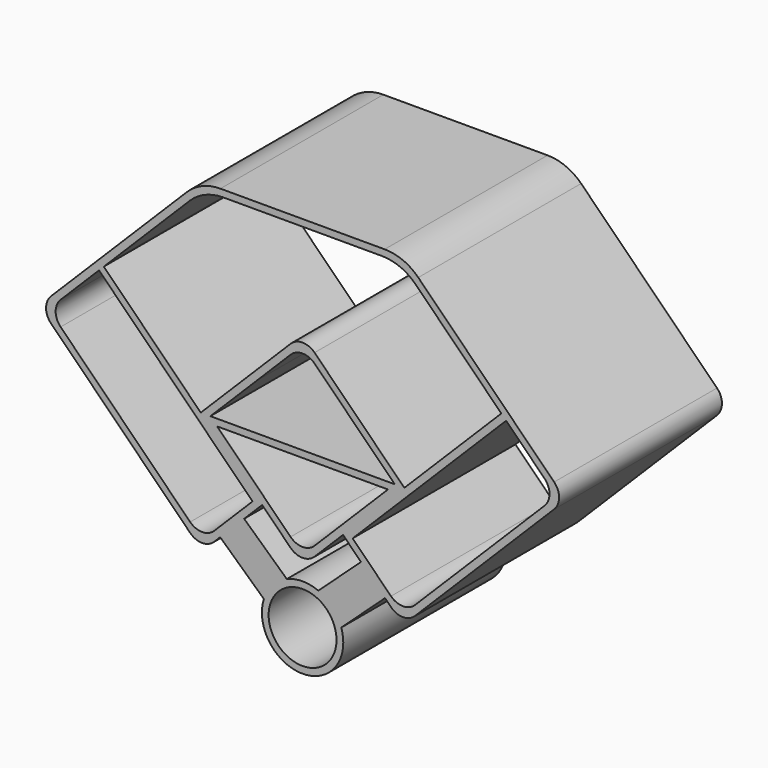
from build123d import *

# Parameters (mm, degrees)
F0_R     = 50
F1_DEPTH = 150


# Not quite as in the source:
# - a feature names something its author has since deleted; it is built from what else it names


with BuildPart() as f1:
    # F0 (on Front) → F1 (new body, symmetric)
    with BuildSketch(Plane.XZ):
        with BuildLine():
            Line((-170.5025253169, 129.4974746831), (-300, 0))
            Line((-300, 0), (-292.9289321881, -7.0710678119))
            Line((-292.9289321881, -7.0710678119), (-285.8578643763, 0))
            Line((-285.8578643763, 0), (-166.3603896932, 119.4974746831))
            ThreePointArc((-166.3603896932, 119.4974746831), (-143.6507552757, 134.6715672758), (-116.8629150102, 140))
            Line((-116.8629150102, 140), (116.8629150102, 140))
            ThreePointArc((116.8629150102, 140), (143.6507552757, 134.6715672758), (166.3603896932, 119.4974746831))
            Line((166.3603896932, 119.4974746831), (285.8578643763, 0))
            Line((285.8578643763, 0), (292.9289321881, -7.0710678119))
            Line((292.9289321881, -7.0710678119), (150, -150))
            Line((150, -150), (59.5836943966, -240.4163056034))
            Line((59.5836943966, -240.4163056034), (86.0845268471, -266.917138054))
            Line((86.0845268471, -266.917138054), (121.4712095943, -302.3038208012))
            Line((121.4712095943, -302.3038208012), (130.2943725152, -311.1269837221))
            ThreePointArc((130.2943725152, -311.1269837221), (147.9720420449, -318.4493141924), (165.6497115746, -311.1269837221))
            Line((165.6497115746, -311.1269837221), (370.7106781187, -106.066017178))
            ThreePointArc((370.7106781187, -106.066017178), (378.033008589, -88.3883476483), (370.7106781187, -70.7106781187))
            Line((370.7106781187, -70.7106781187), (300, 0))
            Line((300, 0), (170.5025253169, 129.4974746831))
            ThreePointArc((170.5025253169, 129.4974746831), (147.7928908994, 144.6715672758), (121.0050506339, 150))
            Line((121.0050506339, 150), (-121.0050506339, 150))
            ThreePointArc((-121.0050506339, 150), (-147.7928908994, 144.6715672758), (-170.5025253169, 129.4974746831))
        make_face()
        with BuildLine():
            Line((73.7258300203, -240.4163056034), (300, -14.1421356237))
            Line((300, -14.1421356237), (356.5685424949, -70.7106781187))
            ThreePointArc((356.5685424949, -70.7106781187), (363.8908729653, -88.3883476483), (356.5685424949, -106.066017178))
            Line((356.5685424949, -106.066017178), (165.6497115746, -296.9848480984))
            ThreePointArc((165.6497115746, -296.9848480984), (147.9720420449, -304.3071785687), (130.2943725152, -296.9848480984))
            Line((130.2943725152, -296.9848480984), (73.7258300203, -240.4163056034))
        make_face(mode=Mode.SUBTRACT)
        with BuildLine():
            Line((-17.6776695297, -17.6776695297), (-150, -150))
            Line((-150, -150), (-59.5836943966, -240.4163056034))
            Line((-59.5836943966, -240.4163056034), (-17.6776695297, -282.3223304703))
            ThreePointArc((-17.6776695297, -282.3223304703), (0, -289.6446609407), (17.6776695297, -282.3223304703))
            Line((17.6776695297, -282.3223304703), (59.5836943966, -240.4163056034))
            Line((59.5836943966, -240.4163056034), (150, -150))
            Line((150, -150), (17.6776695297, -17.6776695297))
            ThreePointArc((17.6776695297, -17.6776695297), (0, -10.3553390593), (-17.6776695297, -17.6776695297))
        make_face()
        with BuildLine():
            ThreePointArc((17.6776695297, -268.1801948466), (0, -275.5025253169), (-17.6776695297, -268.1801948466))
            Line((-17.6776695297, -268.1801948466), (-125.8578643763, -160))
            Line((-125.8578643763, -160), (-135.8578643763, -150))
            Line((-135.8578643763, -150), (-67.9289321881, -82.0710678119))
            Line((-67.9289321881, -82.0710678119), (-17.6776695297, -31.8198051534))
            ThreePointArc((-17.6776695297, -31.8198051534), (0, -24.4974746831), (17.6776695297, -31.8198051534))
            Line((17.6776695297, -31.8198051534), (67.9289321881, -82.0710678119))
            Line((67.9289321881, -82.0710678119), (135.8578643763, -150))
            Line((135.8578643763, -150), (125.8578643763, -160))
            Line((125.8578643763, -160), (17.6776695297, -268.1801948466))
        make_face(mode=Mode.SUBTRACT)
        with BuildLine():
            Line((-292.9289321881, -7.0710678119), (-300, 0))
            Line((-300, 0), (-370.7106781187, -70.7106781187))
            ThreePointArc((-370.7106781187, -70.7106781187), (-378.033008589, -88.3883476483), (-370.7106781187, -106.066017178))
            Line((-370.7106781187, -106.066017178), (-165.6497115746, -311.1269837221))
            ThreePointArc((-165.6497115746, -311.1269837221), (-147.9720420449, -318.4493141924), (-130.2943725152, -311.1269837221))
            Line((-130.2943725152, -311.1269837221), (-121.4712095523, -302.3038207591))
            Line((-121.4712095523, -302.3038207591), (-86.0845268892, -266.917138096))
            Line((-86.0845268892, -266.917138096), (-59.5836943966, -240.4163056034))
            Line((-59.5836943966, -240.4163056034), (-150, -150))
            Line((-150, -150), (-292.9289321881, -7.0710678119))
        make_face()
        with BuildLine():
            Line((-356.5685424949, -70.7106781187), (-300, -14.1421356237))
            Line((-300, -14.1421356237), (-73.7258300203, -240.4163056034))
            Line((-73.7258300203, -240.4163056034), (-130.2943725152, -296.9848480984))
            ThreePointArc((-130.2943725152, -296.9848480984), (-147.9720420449, -304.3071785687), (-165.6497115746, -296.9848480984))
            Line((-165.6497115746, -296.9848480984), (-356.5685424949, -106.066017178))
            ThreePointArc((-356.5685424949, -106.066017178), (-363.8908729653, -88.3883476483), (-356.5685424949, -70.7106781187))
        make_face(mode=Mode.SUBTRACT)
        with BuildLine():
            ThreePointArc((23.2387555319, -324.683089695), (-4.1825e-06, -319.9999946001), (-23.238764161, -324.6830883841))
            ThreePointArc((-23.238764161, -324.6830883841), (-44.1741271353, -339.3964601375), (-57.0750428799, -361.4948561013))
            ThreePointArc((-57.0750428799, -361.4948561013), (-9.3674436165, -439.2642427617), (59.9999941253, -379.9999946001))
            ThreePointArc((59.9999941253, -379.9999946001), (59.264242551, -370.6325585299), (57.0750321743, -361.4948593208))
            ThreePointArc((57.0750321743, -361.4948593208), (44.1741176762, -339.3964626293), (23.2387555319, -324.683089695))
        make_face()
        with Locations((-5.8747e-06, -379.9999946001)):
            Circle(F0_R, mode=Mode.SUBTRACT)
        with BuildLine():
            Line((86.0845268471, -266.917138054), (23.2387555319, -324.683089695))
            ThreePointArc((23.2387555319, -324.683089695), (44.1741176762, -339.3964626293), (57.0750321743, -361.4948593208))
            Line((57.0750321743, -361.4948593208), (121.4712095943, -302.3038208012))
            Line((121.4712095943, -302.3038208012), (86.0845268471, -266.917138054))
        make_face()
        with BuildLine():
            Line((-23.238764161, -324.6830883841), (-86.0845268892, -266.917138096))
            Line((-86.0845268892, -266.917138096), (-121.4712095523, -302.3038207591))
            Line((-121.4712095523, -302.3038207591), (-57.0750428799, -361.4948561013))
            ThreePointArc((-57.0750428799, -361.4948561013), (-44.1741271353, -339.3964601375), (-23.238764161, -324.6830883841))
        make_face()
        Polygon((-135.8578643763, -150), (-125.8578643763, -160), (125.8578643763, -160), (135.8578643763, -150), align=None)
    extrude(amount=F1_DEPTH, both=True)


solid = f1.part
